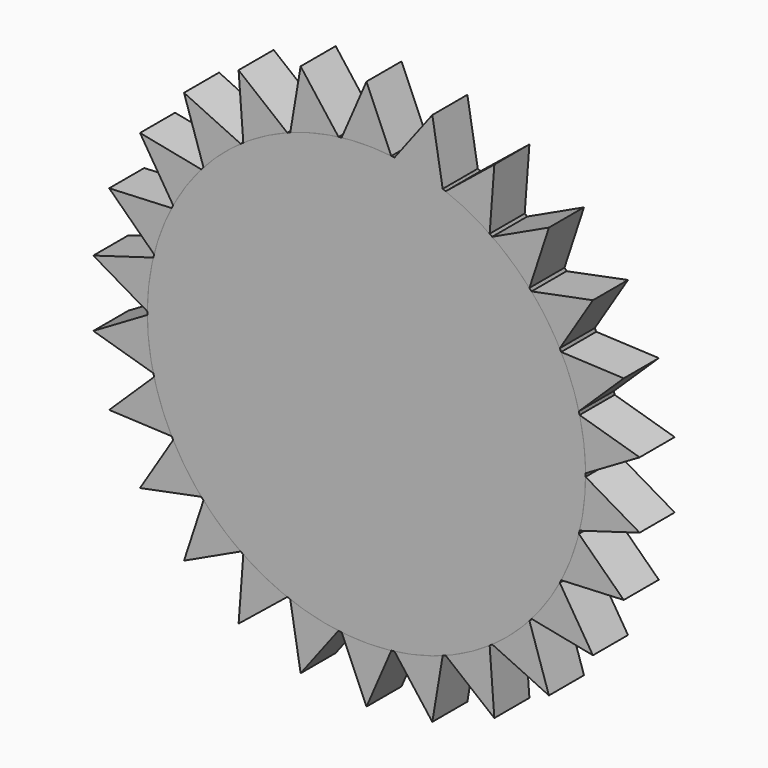
from build123d import *

# Parameters (mm, degrees)
F0_R     = 127
F1_DEPTH = 12.7
F3_DEPTH = 25.4
F4_COUNT = 26


with BuildPart() as f1:
    # F0 (on Front) → F1 (new body, symmetric)
    with BuildSketch(Plane.XZ):
        Circle(F0_R)
    extrude(amount=F1_DEPTH, both=True)

    # F2 (on face) → F3 (join, through all)
    with BuildSketch(Plane.XZ.offset(12.7)):
        with BuildLine():
            Line((0, 159.4720929861), (-14.393243711, 126.1817519908))
            ThreePointArc((-14.393243711, 126.1817519908), (0, 127), (14.393243711, 126.1817519908))
            Line((14.393243711, 126.1817519908), (0, 159.4720929861))
        make_face()
    extrude(amount=-F3_DEPTH)


with BuildPart() as f4_1:
    # F4: instance of F1
    add(f1.part.rotate(Axis((0, 0, 0), (0, -1, 0)), 1 * 360 / F4_COUNT))


with BuildPart() as f4_2:
    # F4: instance of F1
    add(f1.part.rotate(Axis((0, 0, 0), (0, -1, 0)), 2 * 360 / F4_COUNT))


with BuildPart() as f4_3:
    # F4: instance of F1
    add(f1.part.rotate(Axis((0, 0, 0), (0, -1, 0)), 3 * 360 / F4_COUNT))


with BuildPart() as f4_4:
    # F4: instance of F1
    add(f1.part.rotate(Axis((0, 0, 0), (0, -1, 0)), 4 * 360 / F4_COUNT))


with BuildPart() as f4_5:
    # F4: instance of F1
    add(f1.part.rotate(Axis((0, 0, 0), (0, -1, 0)), 5 * 360 / F4_COUNT))


with BuildPart() as f4_6:
    # F4: instance of F1
    add(f1.part.rotate(Axis((0, 0, 0), (0, -1, 0)), 6 * 360 / F4_COUNT))


with BuildPart() as f4_7:
    # F4: instance of F1
    add(f1.part.rotate(Axis((0, 0, 0), (0, -1, 0)), 7 * 360 / F4_COUNT))


with BuildPart() as f4_8:
    # F4: instance of F1
    add(f1.part.rotate(Axis((0, 0, 0), (0, -1, 0)), 8 * 360 / F4_COUNT))


with BuildPart() as f4_9:
    # F4: instance of F1
    add(f1.part.rotate(Axis((0, 0, 0), (0, -1, 0)), 9 * 360 / F4_COUNT))


with BuildPart() as f4_10:
    # F4: instance of F1
    add(f1.part.rotate(Axis((0, 0, 0), (0, -1, 0)), 10 * 360 / F4_COUNT))


with BuildPart() as f4_11:
    # F4: instance of F1
    add(f1.part.rotate(Axis((0, 0, 0), (0, -1, 0)), 11 * 360 / F4_COUNT))


with BuildPart() as f4_12:
    # F4: instance of F1
    add(f1.part.rotate(Axis((0, 0, 0), (0, -1, 0)), 12 * 360 / F4_COUNT))


with BuildPart() as f4_13:
    # F4: instance of F1
    add(f1.part.rotate(Axis((0, 0, 0), (0, -1, 0)), 13 * 360 / F4_COUNT))


with BuildPart() as f4_14:
    # F4: instance of F1
    add(f1.part.rotate(Axis((0, 0, 0), (0, -1, 0)), 14 * 360 / F4_COUNT))


with BuildPart() as f4_15:
    # F4: instance of F1
    add(f1.part.rotate(Axis((0, 0, 0), (0, -1, 0)), 15 * 360 / F4_COUNT))


with BuildPart() as f4_16:
    # F4: instance of F1
    add(f1.part.rotate(Axis((0, 0, 0), (0, -1, 0)), 16 * 360 / F4_COUNT))


with BuildPart() as f4_17:
    # F4: instance of F1
    add(f1.part.rotate(Axis((0, 0, 0), (0, -1, 0)), 17 * 360 / F4_COUNT))


with BuildPart() as f4_18:
    # F4: instance of F1
    add(f1.part.rotate(Axis((0, 0, 0), (0, -1, 0)), 18 * 360 / F4_COUNT))


with BuildPart() as f4_19:
    # F4: instance of F1
    add(f1.part.rotate(Axis((0, 0, 0), (0, -1, 0)), 19 * 360 / F4_COUNT))


with BuildPart() as f4_20:
    # F4: instance of F1
    add(f1.part.rotate(Axis((0, 0, 0), (0, -1, 0)), 20 * 360 / F4_COUNT))


with BuildPart() as f4_21:
    # F4: instance of F1
    add(f1.part.rotate(Axis((0, 0, 0), (0, -1, 0)), 21 * 360 / F4_COUNT))


with BuildPart() as f4_22:
    # F4: instance of F1
    add(f1.part.rotate(Axis((0, 0, 0), (0, -1, 0)), 22 * 360 / F4_COUNT))


with BuildPart() as f4_23:
    # F4: instance of F1
    add(f1.part.rotate(Axis((0, 0, 0), (0, -1, 0)), 23 * 360 / F4_COUNT))


with BuildPart() as f4_24:
    # F4: instance of F1
    add(f1.part.rotate(Axis((0, 0, 0), (0, -1, 0)), 24 * 360 / F4_COUNT))


with BuildPart() as f4_25:
    # F4: instance of F1
    add(f1.part.rotate(Axis((0, 0, 0), (0, -1, 0)), 25 * 360 / F4_COUNT))


solid = Compound([f1.part, f4_1.part, f4_2.part, f4_3.part, f4_4.part, f4_5.part, f4_6.part, f4_7.part, f4_8.part, f4_9.part, f4_10.part, f4_11.part, f4_12.part, f4_13.part, f4_14.part, f4_15.part, f4_16.part, f4_17.part, f4_18.part, f4_19.part, f4_20.part, f4_21.part, f4_22.part, f4_23.part, f4_24.part, f4_25.part])
